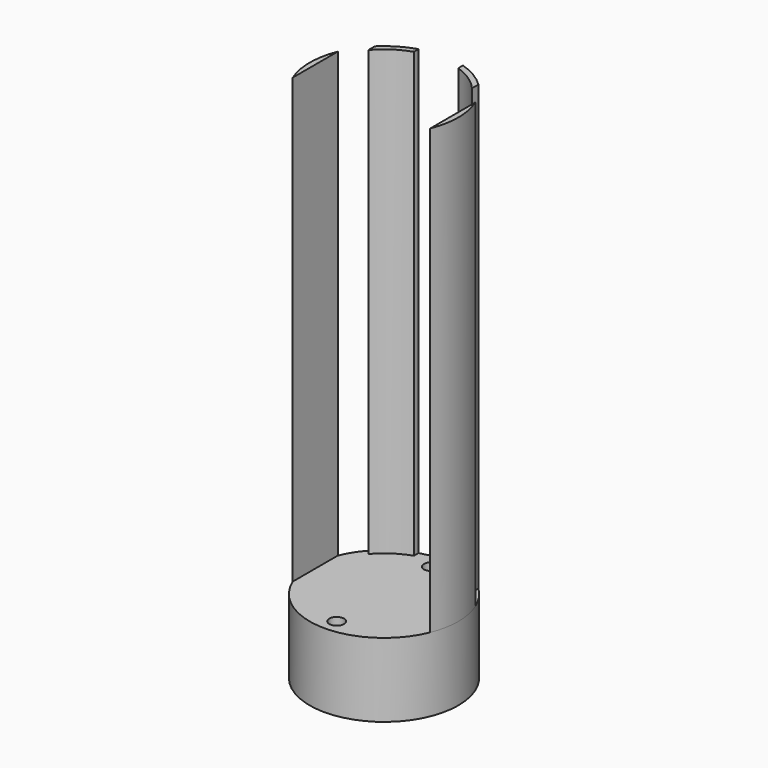
from build123d import *
from build123d import SkipClean  # not in build123d's __all__

# Parameters (mm, degrees)
F1_R     = 12.7635
F1_R_2   = 1.27
F2_DEPTH = 12.7
F3_DEPTH = 76.2


with BuildPart() as f2:
    # F1 (on Top) → F2 (new body)
    with BuildSketch(Plane.XY):
        Circle(F1_R)
        with Locations((0, -10.16)):
            Circle(F1_R_2, mode=Mode.SUBTRACT)
        with Locations((0, 10.16)):
            Circle(F1_R_2, mode=Mode.SUBTRACT)
    extrude(amount=-F2_DEPTH)

    # F0 (on Top) → F3 (join)
    with BuildSketch(Plane.XY):
        with BuildLine():
            Line((-3.81, 11.1796073724), (-3.81, 12.1815775764))
            ThreePointArc((-3.81, 12.1815775764), (-6.5274436814, 10.9681088268), (-8.89, 9.1583203837))
            Line((-8.89, 9.1583203837), (-8.89, 7.7760929135))
            ThreePointArc((-8.89, 7.7760929135), (-6.5740761836, 9.8123006136), (-3.81, 11.1796073724))
        make_face()
        with BuildLine():
            Line((-11.811, -4.8380999628), (-11.811, 4.8380999628))
            ThreePointArc((-11.811, 4.8380999628), (-12.7635, 0), (-11.811, -4.8380999628))
        make_face()
        with BuildLine():
            ThreePointArc((11.811, -4.8380999628), (12.7635, 0), (11.811, 4.8380999628))
            Line((11.811, 4.8380999628), (11.811, -4.8380999628))
        make_face()
        with BuildLine():
            ThreePointArc((8.89, 9.1583203837), (6.5274436814, 10.9681088268), (3.81, 12.1815775764))
            Line((3.81, 12.1815775764), (3.81, 11.1796073724))
            ThreePointArc((3.81, 11.1796073724), (6.5740761836, 9.8123006136), (8.89, 7.7760929135))
            Line((8.89, 7.7760929135), (8.89, 9.1583203837))
        make_face()
    with SkipClean():  # cleaning this boolean's faces spoils the solid; the shape is the same uncleaned
        extrude(amount=F3_DEPTH)


solid = f2.part
